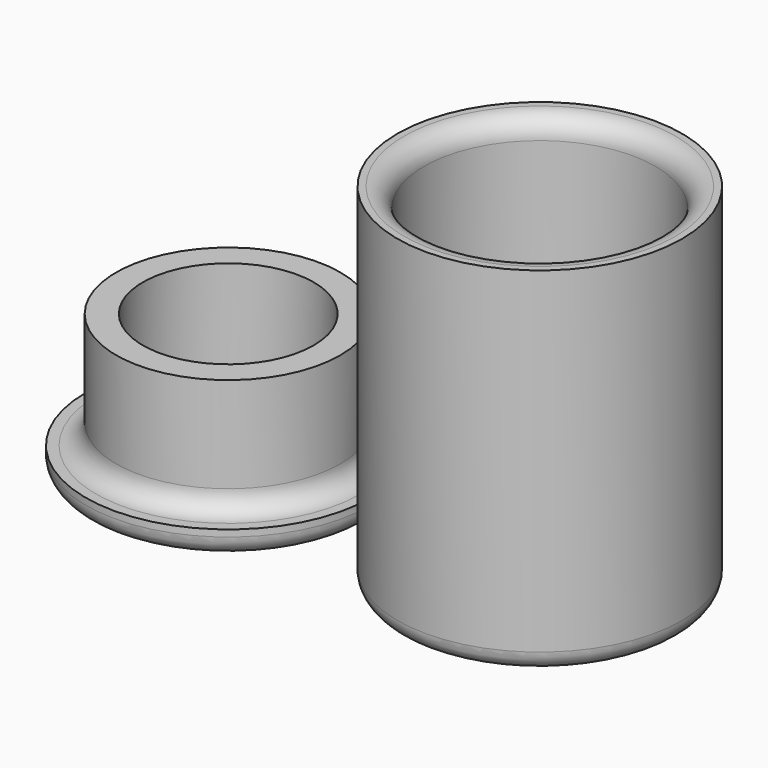
from build123d import *

# Parameters (mm, degrees)
F4_R     = 8
F4_R_2   = 6.5
F4_R_3   = 6.3
F4_R_4   = 4.8
F4_R_5   = 1.275
F5_DEPTH = 1.5
F6_DEPTH = 20
F8_DEPTH = 1.5
F9_DEPTH = 8
F10_R    = 1.125
F10_2_R  = 1.125


with BuildPart() as f5:
    # F4 (on Top) → F5 (new body)
    with BuildSketch(Plane.XY):
        Circle(F4_R)
        Circle(F4_R_2, mode=Mode.SUBTRACT)
        Circle(F4_R_2)
        Circle(F4_R_3, mode=Mode.SUBTRACT)
        Circle(F4_R_3)
        Circle(F4_R_4, mode=Mode.SUBTRACT)
        Circle(F4_R_4)
        Circle(F4_R_5, mode=Mode.SUBTRACT)
    extrude(amount=F5_DEPTH)

    # F4 (on Top) → F6 (join)
    with BuildSketch(Plane.XY):
        Circle(F4_R)
        Circle(F4_R_2, mode=Mode.SUBTRACT)
    extrude(amount=F6_DEPTH)


with BuildPart() as f5_1:
    # F7: moved
    add(f5.part.moved(Location((17.5, 0, 0))))

    # F10
    f10_edges = [f5_1.edges().sort_by_distance(p)[0] for p in [
        (9.5, 0, 0),
        (11, 0, 20),
        (11, 0, 1.5),
    ]]
    fillet(f10_edges, radius=F10_R)


with BuildPart() as f8:
    # F4 (on Top) → F8 (new body)
    with BuildSketch(Plane.XY):
        Circle(F4_R)
        Circle(F4_R_2, mode=Mode.SUBTRACT)
        Circle(F4_R_2)
        Circle(F4_R_3, mode=Mode.SUBTRACT)
        Circle(F4_R_3)
        Circle(F4_R_4, mode=Mode.SUBTRACT)
        Circle(F4_R_4)
        Circle(F4_R_5, mode=Mode.SUBTRACT)
    extrude(amount=F8_DEPTH)

    # F4 (on Top) → F9 (join)
    with BuildSketch(Plane.XY):
        Circle(F4_R_3)
        Circle(F4_R_4, mode=Mode.SUBTRACT)
    extrude(amount=F9_DEPTH)

    # F10#2
    f10_2_edges = [f8.edges().sort_by_distance(p)[0] for p in [
        (-8, 0, 0),
        (-6.3, 0, 1.5),
    ]]
    fillet(f10_2_edges, radius=F10_2_R)


solid = Compound([f5_1.part, f8.part])
